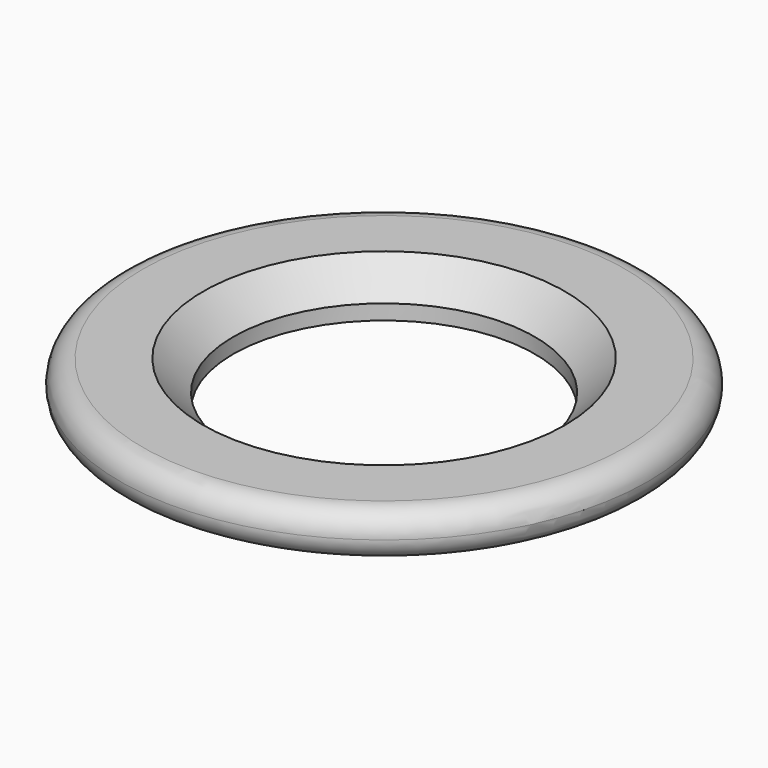
from build123d import *

# Parameters (mm, degrees)
F0_R     = 44.45
F0_R_2   = 25.4
F1_DEPTH = 7.62
F2_SIZE  = 5.08
F3_R     = 3.80999


# Not quite as in the source:
# - a fillet or chamfer is up to 0.001 mm smaller than in the source, because OpenCascade refuses the exact size


with BuildPart() as f1:
    # F0 (on Top) → F1 (new body)
    with BuildSketch(Plane.XY):
        Circle(F0_R)
        Circle(F0_R_2, mode=Mode.SUBTRACT)
    extrude(amount=F1_DEPTH)

    # F2
    f2_edges = [f1.edges().sort_by_distance(p)[0] for p in [
        (-25.4, 0, 7.62),
    ]]
    chamfer(f2_edges, length=F2_SIZE)

    # F3 (radius 3.81 in the source; OpenCascade refuses exactly that, so slightly less here)
    f3_edges = [f1.edges().sort_by_distance(p)[0] for p in [
        (44.45, 0, 3.81),
        (-44.45, 0, 0),
        (-44.45, 0, 7.62),
    ]]
    fillet(f3_edges, radius=F3_R)


solid = f1.part
